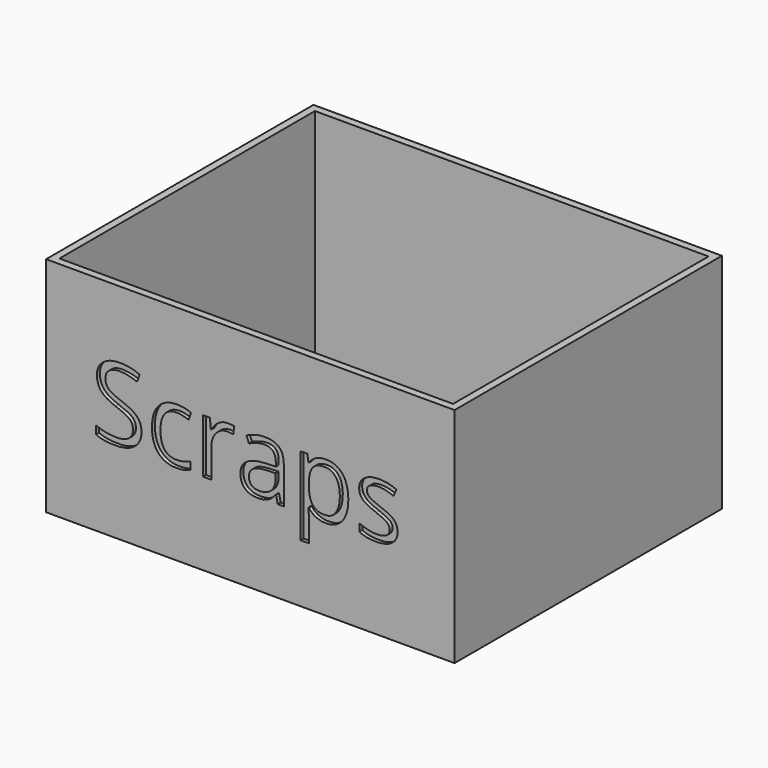
from build123d import *

# Parameters (mm, degrees)
F0_W         = 110
F0_H         = 90
F0_W_2       = 106
F0_H_2       = 86
F1_DEPTH     = 1
F2_DEPTH     = 60
F3_TEXT_SIZE = 27.2347358987
F4_DEPTH     = 1


# Not quite as in the source:
# - Text() gives the source's letters only with a copy of the font that has no kerning and outlines rounded to 1/6400 em; it was checked with that copy


with BuildPart() as f1:
    # F0 (on Top) → F1 (new body)
    with BuildSketch(Plane.XY):
        Rectangle(F0_W, F0_H)
        Rectangle(F0_W_2, F0_H_2, mode=Mode.SUBTRACT)
        Rectangle(F0_W_2, F0_H_2)
    extrude(amount=F1_DEPTH)


with BuildPart() as f2:
    # F0 (on Top) → F2 (new body)
    with BuildSketch(Plane.XY):
        Rectangle(F0_W, F0_H)
        Rectangle(F0_W_2, F0_H_2, mode=Mode.SUBTRACT)
    extrude(amount=F2_DEPTH)

    # F3 (on face) → F4 (cut)
    with BuildSketch(Plane.XZ.offset(45)):
        with Locations((-42.9624691606, 22.189611569)):
            Text('Scraps', F3_TEXT_SIZE, font='Open Sans', text_align=(TextAlign.LEFT, TextAlign.BOTTOM))
    extrude(amount=-F4_DEPTH, mode=Mode.SUBTRACT)


solid = Compound([f1.part, f2.part])
